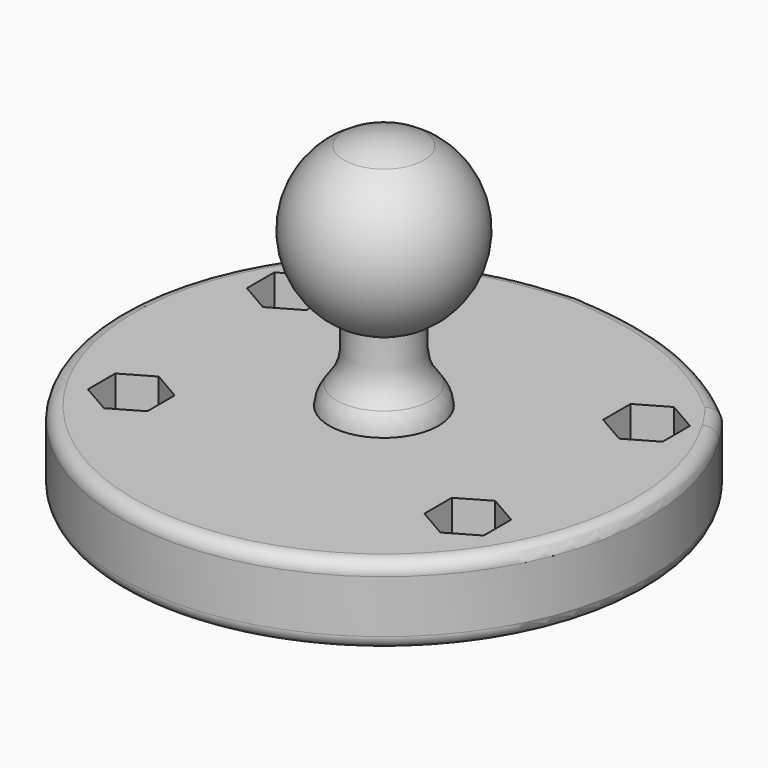
from build123d import *

# Parameters (mm, degrees)
F0_R     = 2.5
F1_DEPTH = 12
F3_R     = 2.5
F4_DEPTH = 6
F8_R     = 2


# Not quite as in the source:
# - a fillet or chamfer that OpenCascade refuses, or shapes differently, is made with other operations: its cross-section is extruded or revolved along the edge and cut away or added


with BuildPart() as f1:
    # F0 (on Top) → F1 (new body)
    with BuildSketch(Plane.XY):
        with BuildLine():
            ThreePointArc((-31.3651592039, 24.7400687451), (-33.0304528025, 22.4689333996), (-34.5318159842, 20.0862527403))
            ThreePointArc((-34.5318159842, 20.0862527403), (0.3556410553, -40.0322385106), (34.289361103, 20.6296959515))
            ThreePointArc((34.289361103, 20.6296959515), (32.9313235996, 22.7293613836), (31.4447447441, 24.7400687451))
            add(Edge.make_bspline(
                [(31.4447447441, 24.7400687451), (22.988602022, 32.1085255021), (13.1297165658, 36.2919575894), (0.0397927701, 36.9132596428)],
                knots=[0, 0, 0, 0, 0.5, 0.5, 0.5, 0.5], degree=3))
            add(Edge.make_bspline(
                [(-31.3651592039, 24.7400687451), (-22.9090164817, 32.1085255021), (-13.0501310255, 36.2919575894), (0.0397927701, 36.9132596428)],
                knots=[0, 0, 0, 0, 0.5, 0.5, 0.5, 0.5], degree=3))
        make_face()
        with Locations((-25.4602072299, -16.0334855318)):
            Circle(F0_R, mode=Mode.SUBTRACT)
        with Locations((25.5397927701, -16.0334855318)):
            Circle(F0_R, mode=Mode.SUBTRACT)
        with Locations((-26.9602072299, 15.9665144682)):
            Circle(F0_R, mode=Mode.SUBTRACT)
        with Locations((27.0397927701, 15.9665144682)):
            Circle(F0_R, mode=Mode.SUBTRACT)
    extrude(amount=F1_DEPTH)

    # F3 (on face) → F4 (cut)
    with BuildSketch(Plane.XY.offset(12)):
        Polygon((-22.4602072299, 13.3684382568), (-22.4602072299, 18.5645906795), (-26.9602072299, 21.1626668909), (-31.4602072299, 18.5645906795), (-31.4602072299, 13.3684382568), (-26.9602072299, 10.7703620455), align=None)
        with Locations((-26.9602072299, 15.9665144682)):
            Circle(F3_R, mode=Mode.SUBTRACT)
        Polygon((22.5397927701, 18.5645906795), (22.5397927701, 13.3684382568), (27.0397927701, 10.7703620455), (31.5397927701, 13.3684382568), (31.5397927701, 18.5645906795), (27.0397927701, 21.1626668909), align=None)
        with Locations((27.0397927701, 15.9665144682)):
            Circle(F3_R, mode=Mode.SUBTRACT)
        Polygon((21.0397927701, -13.4354093205), (21.0397927701, -18.6315617432), (25.5397927701, -21.2296379545), (30.0397927701, -18.6315617432), (30.0397927701, -13.4354093205), (25.5397927701, -10.8373331091), align=None)
        with Locations((25.5397927701, -16.0334855318)):
            Circle(F3_R, mode=Mode.SUBTRACT)
        Polygon((-20.9602072299, -18.6315617432), (-20.9602072299, -13.4354093205), (-25.4602072299, -10.8373331091), (-29.9602072299, -13.4354093205), (-29.9602072299, -18.6315617432), (-25.4602072299, -21.2296379545), align=None)
        with Locations((-25.4602072299, -16.0334855318)):
            Circle(F3_R, mode=Mode.SUBTRACT)
    extrude(amount=-F4_DEPTH, mode=Mode.SUBTRACT)

    # F5 (on Front) → F6 (revolve)
    with BuildSketch(Plane.XZ):
        with BuildLine():
            Line((-8.284470181, 11.8907699668), (0, 11.8907699668))
            Line((0, 11.8907699668), (0, 48.1916638966))
            ThreePointArc((0, 48.1916638966), (-3.1039423325, 47.8080717015), (-6.0211163429, 46.6803763667))
            ThreePointArc((-6.0211163429, 46.6803763667), (-12.7413209188, 34.9713010104), (-5.1760724611, 23.7895922406))
            add(Edge.make_bspline(
                [(-8.284470181, 13.6864552548), (-7.2384952575, 14.7658121918), (-4.9346184441, 17.14342214), (-5.0921300249, 21.4398414936), (-5.1760724611, 23.7895922406)],
                knots=[0, 0, 0, 0, 0.4540341601, 1, 1, 1, 1], degree=3))
            Line((-8.284470181, 13.6864552548), (-8.284470181, 11.8907699668))
        make_face()
    revolve(axis=Axis((0, 0, 50.5361706018), (0, 0, 1)))

    # F7: fillet of radius 5 on 1 edges, made by hand

    # F7_s1 → F7_t2 (revolve, cut)
    with BuildSketch(Plane.XZ):
        with BuildLine():
            ThreePointArc((-8.284470181, 12), (-7.9344186734, 13.5789038819), (-7.0987068449, 14.9634829753))
            Line((-7.0987068449, 14.9634829753), (-7.1748362782, 15.0283236215))
            ThreePointArc((-7.1748362782, 15.0283236215), (-7.7543234481, 14.3838527889), (-8.3562826351, 13.7560467158))
            Line((-8.3562826351, 13.7560467158), (-8.384470181, 13.6864552548))
            ThreePointArc((-8.384470181, 13.6864552548), (-8.384470181, 12.8432276274), (-8.384314881, 12.0055709867))
            Line((-8.384314881, 12.0055709867), (-8.284470181, 12))
        make_face()
    revolve(axis=Axis((0, 0, 13.6864552548), (0, 0, 1)), mode=Mode.SUBTRACT)

    # F8
    f8_edges = [f1.edges().sort_by_distance(p)[0] for p in [
        (-2.459557, -39.955325, 12),
        (-2.459557, -39.955325, 0),
        (16.831403, 33.608309, 12),
        (-16.751817, 33.608309, 12),
        (-16.751817, 33.608309, 0),
        (16.831403, 33.608309, 0),
    ]]
    fillet(f8_edges, radius=F8_R)


solid = f1.part
